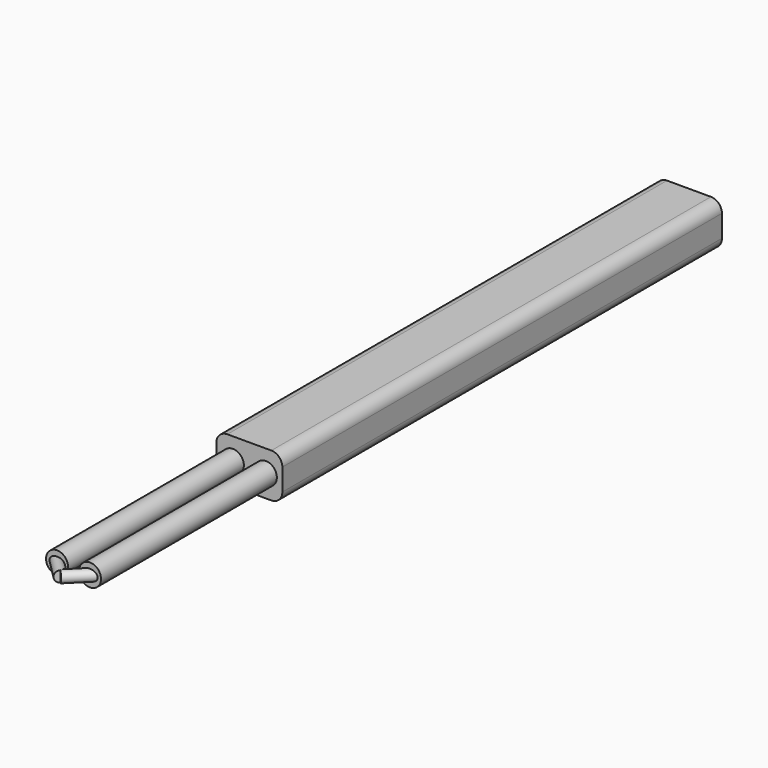
from build123d import *

# Parameters (mm, degrees)
F1_DEPTH      = 25
F2_R          = 0.5
F3_DEPTH      = 10
F6_R          = 0.25
F7_DEPTH      = 0.3
F7_DEPTH_BACK = 1.0606601718


# Not quite as in the source:
# - the program builds the solid bodies; features that only make, move or delete a surface that nothing else refers to are left out


with BuildPart() as f1:
    # F0 (on Front) → F1 (new body)
    with BuildSketch(Plane.XZ):
        with BuildLine():
            Line((-1, -1), (1, -1))
            ThreePointArc((1, -1), (1.3535533906, -0.8535533906), (1.5, -0.5))
            Line((1.5, -0.5), (1.5, 0.5))
            ThreePointArc((1.5, 0.5), (1.3535533906, 0.8535533906), (1, 1))
            Line((1, 1), (-1, 1))
            ThreePointArc((-1, 1), (-1.3535533906, 0.8535533906), (-1.5, 0.5))
            Line((-1.5, 0.5), (-1.5, -0.5))
            ThreePointArc((-1.5, -0.5), (-1.3535533906, -0.8535533906), (-1, -1))
        make_face()
    extrude(amount=F1_DEPTH)


with BuildPart() as f3:
    # F2 (on face) → F3 (new body)
    with BuildSketch(Plane.XZ.offset(25)):
        with Locations((-0.75, 0)):
            Circle(F2_R)
    extrude(amount=F3_DEPTH)


with BuildPart() as f3b:
    # F2 (on face) → F3, piece 2 (new body)
    with BuildSketch(Plane.XZ.offset(25)):
        with Locations((0.75, 0)):
            Circle(F2_R)
    extrude(amount=F3_DEPTH)


with BuildPart() as f7:
    # F6 (on face) → F7 (new body, two sides)
    with BuildSketch(Plane(origin=(-17.125, -17.125, 0), x_dir=(-0.7071067812, 0.7071067812, 0), z_dir=(0.7071067812, 0.7071067812, 0))) as f7_sk:
        with Locations((-25.2743531018, 0)):
            Circle(F6_R)
    extrude(amount=F7_DEPTH)
    extrude(f7_sk.sketch, amount=-F7_DEPTH_BACK)


with BuildPart() as f8_1:
    # F8: instance of F7
    add(f7.part.mirror(Plane.YZ))


solid = Compound([f1.part, f3.part, f3b.part, f7.part, f8_1.part])
